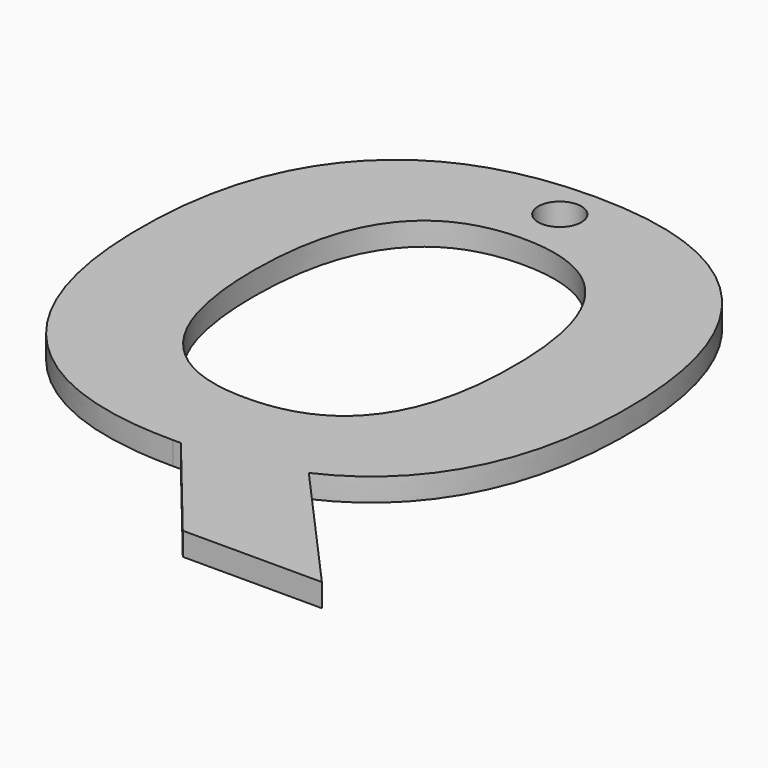
from build123d import *

# Parameters (mm, degrees)
F0_TEXT_SIZE = 63.2898578937
F1_DEPTH     = 2.032
F2_R         = 1.905
F3_DEPTH     = 2.0330001


# Not quite as in the source:
# - Text() gives the source's letters only with a copy of the font that has no kerning and outlines rounded to 1/6400 em; it was checked with that copy


with BuildPart() as f1:
    # F0 (on Top) → F1 (new body)
    with BuildSketch(Plane.XY):
        with Locations((-22.7843488417, -23.4945250283)):
            Text('Q', F0_TEXT_SIZE, font='Open Sans', font_style=FontStyle.BOLD, text_align=(TextAlign.LEFT, TextAlign.BOTTOM))
    extrude(amount=F1_DEPTH)

    # F2 (on face) → F3 (cut, through all)
    with BuildSketch(Plane.XY.offset(2.032)):
        with Locations((2.1860681009, 18.8310984522)):
            Circle(F2_R)
    extrude(amount=-F3_DEPTH, mode=Mode.SUBTRACT)


solid = f1.part
